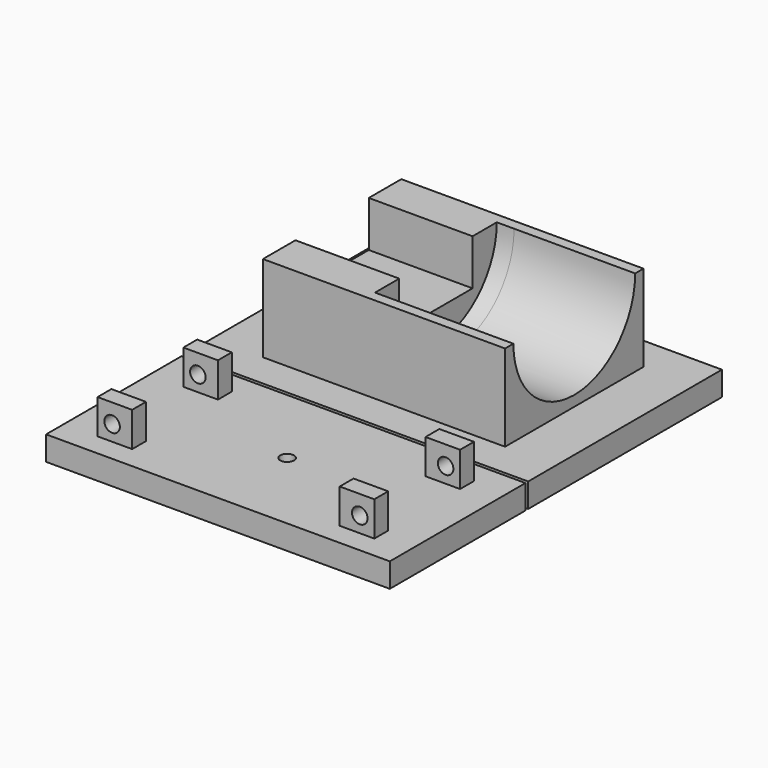
from build123d import *

# Parameters (mm, degrees)
F0_W          = 99.3576076057
F0_H          = 120
F0_R          = 2
F1_DEPTH      = 7
F2_W          = 70
F2_H          = 50
F2_R          = 2
F3_DEPTH      = 25
F2_W_2        = 10
F2_H_2        = 5
F4_DEPTH      = 10
F5_R          = 22
F6_DEPTH      = 35
F6_DEPTH_BACK = 5
F7_W          = 26.5
F7_H          = 26.5
F8_DEPTH      = 30
F9_R          = 2.25
F10_DEPTH     = 40
F11_W         = 99.3576076057
F11_H         = 1
F12_DEPTH     = 25


# Not quite as in the source:
# - a feature names something its author has since deleted; it is built from what else it names


with BuildPart() as f1:
    # F0 (on Top) → F1 (new body)
    with BuildSketch(Plane.XY):
        Rectangle(F0_W, F0_H)
        with Locations((0, -35)):
            Circle(F0_R, mode=Mode.SUBTRACT)
        with Locations((0, 25)):
            Circle(F0_R, mode=Mode.SUBTRACT)
    extrude(amount=-F1_DEPTH)

    # F2 (on face) → F3 (join)
    with BuildSketch(Plane.XY):
        with Locations((0, 25)):
            Rectangle(F2_W, F2_H)
        with Locations((0, 25)):
            Circle(F2_R, mode=Mode.SUBTRACT)
    extrude(amount=F3_DEPTH)

    # F2 (on face) → F4 (join)
    with BuildSketch(Plane.XY):
        with Locations((0, 25)):
            Rectangle(F2_W, F2_H)
        with Locations((0, 25)):
            Circle(F2_R, mode=Mode.SUBTRACT)
        with Locations((-35, -20)):
            Rectangle(F2_W_2, F2_H_2)
        with Locations((35, -51)):
            Rectangle(F2_W_2, F2_H_2)
        with Locations((-35, -51)):
            Rectangle(F2_W_2, F2_H_2)
        with Locations((35, -20)):
            Rectangle(F2_W_2, F2_H_2)
    extrude(amount=F4_DEPTH)

    # F5 (on Right) → F6 (cut, two sides)
    with BuildSketch(Plane.YZ) as f6_sk:
        with Locations((25, 25)):
            Circle(F5_R)
    extrude(amount=F6_DEPTH, mode=Mode.SUBTRACT)
    extrude(f6_sk.sketch, amount=-F6_DEPTH_BACK, mode=Mode.SUBTRACT)

    # F7 (on face) → F8 (cut)
    with BuildSketch(Plane(origin=(-35, 0, 0), x_dir=(0, -1, 0), z_dir=(-1, 0, 0))):
        with Locations((-25, 25)):
            Rectangle(F7_W, F7_H)
    extrude(amount=-F8_DEPTH, mode=Mode.SUBTRACT)

    # F9 (on face) → F10 (cut)
    with BuildSketch(Plane.XZ.offset(53.5)):
        with Locations((35.8, 4.5)):
            Circle(F9_R)
        with Locations((-35.8, 4.5)):
            Circle(F9_R)
    extrude(amount=-F10_DEPTH, mode=Mode.SUBTRACT)

    # F11 (on face) → F12 (cut)
    with BuildSketch(Plane(origin=(0, 0, -7), x_dir=(1, 0, 0), z_dir=(0, 0, -1))):
        with Locations((0, 10.5)):
            Rectangle(F11_W, F11_H)
    extrude(amount=-F12_DEPTH, mode=Mode.SUBTRACT)


solid = f1.part
